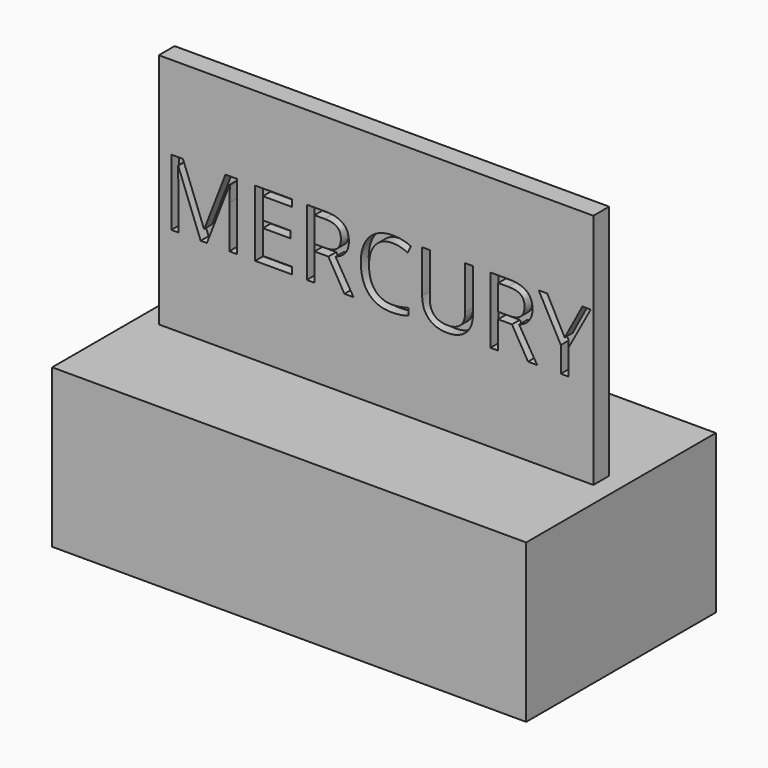
from build123d import *

# Parameters (mm, degrees)
F0_W         = 152.4
F0_H         = 76.2
F1_DEPTH     = 50.8
F2_W         = 139.7
F2_H         = 6.35
F3_DEPTH     = 76.2
F5_TEXT_SIZE = 29.8574052429
F6_DEPTH     = 3.175
F7_TEXT_SIZE = 4.9668139513
F8_DEPTH     = 1.27
F9_W         = 5.08
F9_H         = 3.81
F10_DEPTH    = 2.54


# Not quite as in the source:
# - Text() gives the source's letters only with a copy of the font that has no kerning and outlines rounded to 1/6400 em; it was checked with that copy


with BuildPart() as f1:
    # F0 (on Top) → F1 (new body)
    with BuildSketch(Plane.XY):
        Rectangle(F0_W, F0_H)
    extrude(amount=F1_DEPTH)

    # F2 (on face) → F3 (join)
    with BuildSketch(Plane.XY.offset(50.8)):
        Rectangle(F2_W, F2_H)
    extrude(amount=F3_DEPTH)

    # F5 (on face) → F6 (cut)
    with BuildSketch(Plane.XZ.offset(3.175)):
        with Locations((-68.758700043, 78.867)):
            Text('MERCURY', F5_TEXT_SIZE, font='Open Sans', text_align=(TextAlign.LEFT, TextAlign.BOTTOM))
    extrude(amount=-F6_DEPTH, mode=Mode.SUBTRACT)

    # F7 (on face) → F8 (cut, symmetric)
    with BuildSketch(Plane(origin=(0, 38.1, 0), x_dir=(-1, 0, 0), z_dir=(0, 1, 0))):
        with Locations((57.7675962214, 0)):
            Text('On/Off', F7_TEXT_SIZE, font='Open Sans', text_align=(TextAlign.LEFT, TextAlign.BOTTOM))
    extrude(amount=F8_DEPTH, both=True, mode=Mode.SUBTRACT)

    # F9 (on face) → F10 (join)
    with BuildSketch(Plane(origin=(0, 38.1, 0), x_dir=(-1, 0, 0), z_dir=(0, 1, 0))):
        with Locations((62.0614809394, 7.0280198947)):
            Rectangle(F9_W, F9_H)
        with Locations((69.7347519612, 7.0165816459)):
            Rectangle(F9_W, F9_H)
    extrude(amount=F10_DEPTH)


solid = f1.part
